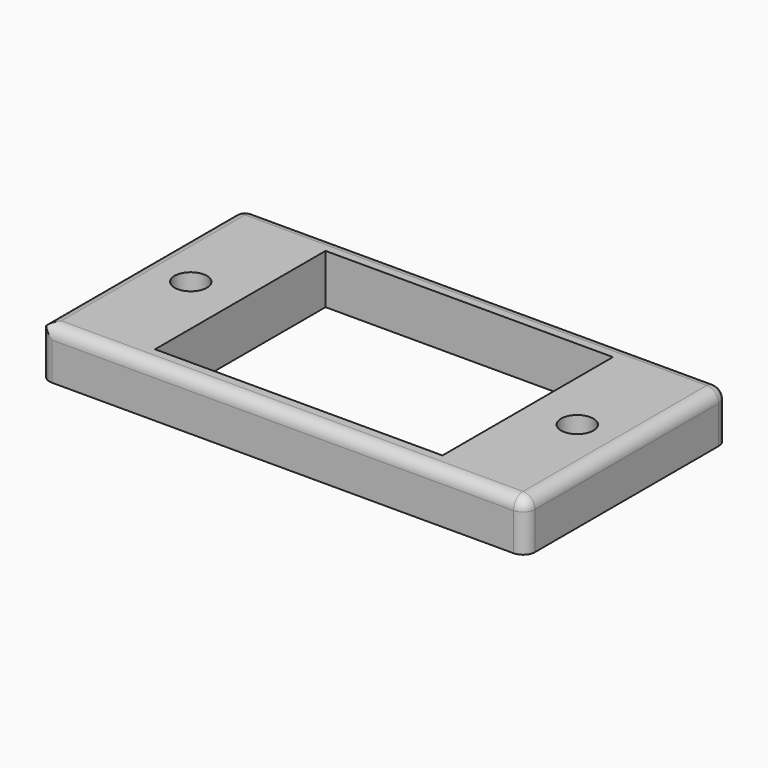
from build123d import *

# Parameters (mm, degrees)
F0_W         = 49
F0_H         = 25.5652221807
F1_DEPTH     = 5
F3_D         = 3.2639
F4_W         = 29
F4_H         = 21.5
F5_DEPTH     = 25
F7_R         = 1.207
F8_R         = 1.207
F9_T1_DEPTH  = 6.8105
F9_T3_DEPTH  = 27.3757221807
F9_T6_ANGLE  = 90
F9_T7_DEPTH  = 9.828
F9_T9_DEPTH  = 49.6035
F9_T11_DEPTH = 6.8105
F9_T14_ANGLE = 90


# Not quite as in the source:
# - a fillet or chamfer that OpenCascade refuses, or shapes differently, is made with other operations: its cross-section is extruded or revolved along the edge and cut away or added
# - a feature of the source that left no trace in its solid (it failed there, or was rolled back) is left out


with BuildPart() as f1:
    # F0 (on Top) → F1 (new body)
    with BuildSketch(Plane.XY):
        Rectangle(F0_W, F0_H)
    extrude(amount=-F1_DEPTH)

    # F3 (through all)
    with Locations(Plane.XY):
        with Locations((-19.5, 0), (19.5, 0)):
            Hole(F3_D / 2)

    # F4 (on Top) → F5 (cut)
    with BuildSketch(Plane.XY):
        Rectangle(F4_W, F4_H)
    extrude(amount=-F5_DEPTH, mode=Mode.SUBTRACT)

    # F7
    f7_edges = [f1.edges().sort_by_distance(p)[0] for p in [
        (0, 12.782611, 0),
    ]]
    fillet(f7_edges, radius=F7_R)

    # F8
    f8_edges = [f1.edges().sort_by_distance(p)[0] for p in [
        (24.5, -0.6035, 0),
    ]]
    fillet(f8_edges, radius=F8_R)

    # F9: fillet of radius 1.207 on 7 edges, made by hand

    # F9_s2 → F9_t1 (cut)
    with BuildSketch(Plane.XY.offset(-8.0175)):
        with BuildLine():
            ThreePointArc((-23.293, 12.7826110903), (-24.1464778849, 12.4290889752), (-24.5, 11.5756110903))
            Line((-24.5, 11.5756110903), (-24.5, 12.7826110903))
            Line((-24.5, 12.7826110903), (-23.293, 12.7826110903))
        make_face()
    extrude(amount=F9_T1_DEPTH, mode=Mode.SUBTRACT)

    # F9_s4 → F9_t3 (cut)
    with BuildSketch(Plane.XZ.offset(-11.5756110903)):
        with BuildLine():
            ThreePointArc((-24.5, -1.207), (-24.1464778849, -0.3535221151), (-23.293, 0))
            Line((-23.293, 0), (-24.5, 0))
            Line((-24.5, 0), (-24.5, -1.207))
        make_face()
    extrude(amount=F9_T3_DEPTH, mode=Mode.SUBTRACT)

    # F9_s5 → F9_t6 (revolve, cut)
    with BuildSketch(Plane.XY.offset(-1.207)):
        with BuildLine():
            ThreePointArc((-23.293, 12.7826110903), (-24.1464778849, 12.4290889752), (-24.5, 11.5756110903))
            Line((-24.5, 11.5756110903), (-24.5, 12.7826110903))
            Line((-24.5, 12.7826110903), (-23.293, 12.7826110903))
        make_face()
    revolve(axis=Axis((-24.5, 11.5756110903, -1.207), (1, 0, 0)), revolution_arc=F9_T6_ANGLE, mode=Mode.SUBTRACT)

    # F9_s8 → F9_t7 (cut)
    with BuildSketch(Plane.XY.offset(-8.0175)):
        with BuildLine():
            ThreePointArc((-24.5, -11.5756110903), (-24.1464778849, -12.4290889752), (-23.293, -12.7826110903))
            Line((-23.293, -12.7826110903), (-24.5, -12.7826110903))
            Line((-24.5, -12.7826110903), (-24.5, -11.5756110903))
        make_face()
    extrude(amount=F9_T7_DEPTH, mode=Mode.SUBTRACT)

    # F9_s10 → F9_t9 (cut)
    with BuildSketch(Plane.YZ.offset(-26.3105)):
        with BuildLine():
            ThreePointArc((-11.5756110903, 0), (-12.4290889752, -0.3535221151), (-12.7826110903, -1.207))
            Line((-12.7826110903, -1.207), (-12.7826110903, 0))
            Line((-12.7826110903, 0), (-11.5756110903, 0))
        make_face()
    extrude(amount=F9_T9_DEPTH, mode=Mode.SUBTRACT)

    # F9_s12 → F9_t11 (cut)
    with BuildSketch(Plane.XY.offset(-8.0175)):
        with BuildLine():
            ThreePointArc((24.5, -11.5756110903), (24.1464778849, -12.4290889752), (23.293, -12.7826110903))
            Line((23.293, -12.7826110903), (24.5, -12.7826110903))
            Line((24.5, -12.7826110903), (24.5, -11.5756110903))
        make_face()
    extrude(amount=F9_T11_DEPTH, mode=Mode.SUBTRACT)

    # F9_s13 → F9_t14 (revolve, cut)
    with BuildSketch(Plane.XY.offset(-1.207)):
        with BuildLine():
            ThreePointArc((23.293, -12.7826110903), (24.1464778849, -12.4290889752), (24.5, -11.5756110903))
            Line((24.5, -11.5756110903), (24.5, -12.7826110903))
            Line((24.5, -12.7826110903), (23.293, -12.7826110903))
        make_face()
    revolve(axis=Axis((23.293, -12.7826110903, -1.207), (0, -1, 0)), revolution_arc=F9_T14_ANGLE, mode=Mode.SUBTRACT)


solid = f1.part
